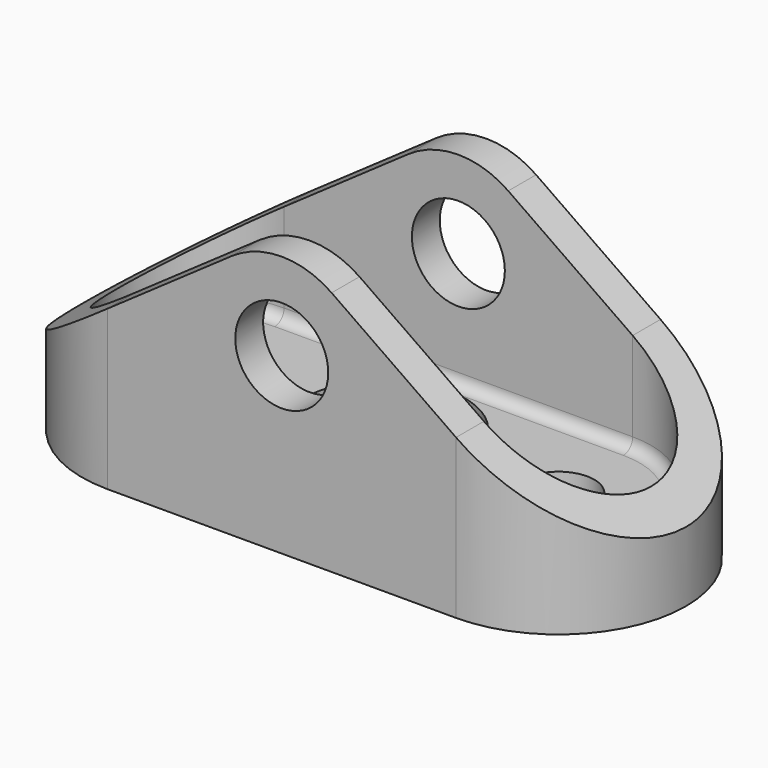
from build123d import *

# Parameters (mm, degrees)
F0_R     = 3.0896655398
F1_DEPTH = 25
F2_R     = 4
F3_DEPTH = 25
F6_DEPTH = 25
F7_R     = 0.99999


# Not quite as in the source:
# - a fillet or chamfer is up to 0.001 mm smaller than in the source, because OpenCascade refuses the exact size


with BuildPart() as f1:
    # F0 (on Top) → F1 (new body)
    with BuildSketch(Plane.XY):
        with BuildLine():
            ThreePointArc((-15, 11), (-26, 0), (-15, -11))
            Line((-15, -11), (15, -11))
            ThreePointArc((15, -11), (26, 0), (15, 11))
            Line((15, 11), (-15, 11))
        make_face()
        with Locations((-15, 0)):
            Circle(F0_R, mode=Mode.SUBTRACT)
        with BuildLine():
            ThreePointArc((7, 0), (0, -7), (-7, 0))
            ThreePointArc((-7, 0), (0, 7), (7, 0))
        make_face(mode=Mode.SUBTRACT)
        with BuildLine():
            ThreePointArc((18.1, 0), (15, -3.1), (11.9, 0))
            ThreePointArc((11.9, 0), (15, 3.1), (18.1, 0))
        make_face(mode=Mode.SUBTRACT)
    extrude(amount=F1_DEPTH)

    # F2 (on face) → F3 (cut)
    with BuildSketch(Plane.XZ.offset(11)):
        with BuildLine():
            Line((15, 25), (-15, 25))
            Line((-15, 25), (-15, 13.6771502157))
            Line((-15, 13.6771502157), (-4.2923891696, 21.1502353789))
            ThreePointArc((-4.2923891696, 21.1502353789), (0, 22.5), (4.2923891696, 21.1502353789))
            Line((4.2923891696, 21.1502353789), (15, 13.6771502157))
            Line((15, 13.6771502157), (15, 25))
        make_face()
        with BuildLine():
            Line((26, 25), (-26, 25))
            Line((-26, 25), (-26, 6))
            Line((-26, 6), (-4.2923891696, 21.1502353789))
            ThreePointArc((-4.2923891696, 21.1502353789), (0, 22.5), (4.2923891696, 21.1502353789))
            Line((4.2923891696, 21.1502353789), (26, 6))
            Line((26, 6), (26, 25))
        make_face()
        with Locations((0, 15)):
            Circle(F2_R)
    extrude(amount=-F3_DEPTH, mode=Mode.SUBTRACT)

    # F5 (on offset) → F6 (cut)
    with BuildSketch(Plane(origin=(0, 0, 5), x_dir=(1, 0, 0), z_dir=(0, 0, -1))):
        with BuildLine():
            Line((-15, -8), (15, -8))
            ThreePointArc((15, -8), (23, 0), (15, 8))
            Line((15, 8), (-15, 8))
            ThreePointArc((-15, 8), (-23, 0), (-15, -8))
        make_face()
    extrude(amount=-F6_DEPTH, mode=Mode.SUBTRACT)

    # F7 (radius 1 in the source; OpenCascade refuses exactly that, so slightly less here)
    f7_edges = [f1.edges().sort_by_distance(p)[0] for p in [
        (0, -8, 5),
    ]]
    fillet(f7_edges, radius=F7_R)


solid = f1.part
